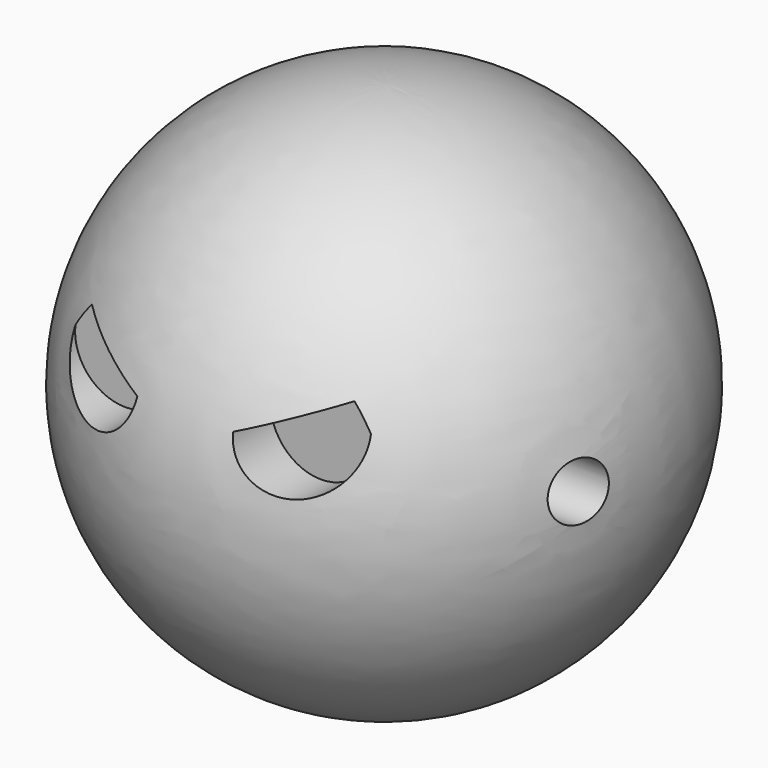
from build123d import *

# Parameters (mm, degrees)
F5_DEPTH = 13.97
F6_R     = 1.6
F7_DEPTH = 15.24
F8_W     = 36.1250601709
F8_H     = 9.7824148252
F9_DEPTH = 76.2


# Not quite as in the source:
# - ends of sketch curves that miss each other by under 0.0002 mm in the source are joined


with BuildPart() as f1:
    # F0 (on Front) → F1 (revolve)
    with BuildSketch(Plane.XZ):
        with BuildLine():
            Line((0, 30), (0, 0))
            ThreePointArc((0, 0), (15.0000006192, 15), (0, 30))
        make_face()
    revolve(axis=Axis((0, 0, 15), (0, 0, 1)))

    # F4 (on offset) → F5 (cut)
    with BuildSketch(Plane.XZ.offset(25.4)):
        with BuildLine():
            ThreePointArc((-7.7757835388, 21.3449876755), (-6.6607308484, 16.8981042804), (-2.7180244215, 19.2375872284))
            Line((-2.7180244215, 19.2375872284), (-7.7757835388, 21.3449876755))
        make_face()
        with BuildLine():
            Line((7.7757835388, 21.3449876755), (2.7180244215, 19.2375872284))
            ThreePointArc((2.7180244215, 19.2375872284), (6.6607308484, 16.8981042804), (7.7757835388, 21.3449876755))
        make_face()
    extrude(amount=-F5_DEPTH, mode=Mode.SUBTRACT)

    # F6 (on offset) → F7 (cut)
    with BuildSketch(Plane.YZ.offset(25.4)):
        with Locations((-4.0855947882, 15.938160941)):
            Circle(F6_R)
    extrude(amount=-F7_DEPTH, mode=Mode.SUBTRACT)

    # F8 (on offset) → F9 (cut)
    with BuildSketch(Plane.XZ.offset(25.4)):
        with Locations((1.2260917574, -4.0021650784)):
            Rectangle(F8_W, F8_H)
    extrude(amount=-F9_DEPTH, mode=Mode.SUBTRACT)


solid = f1.part
